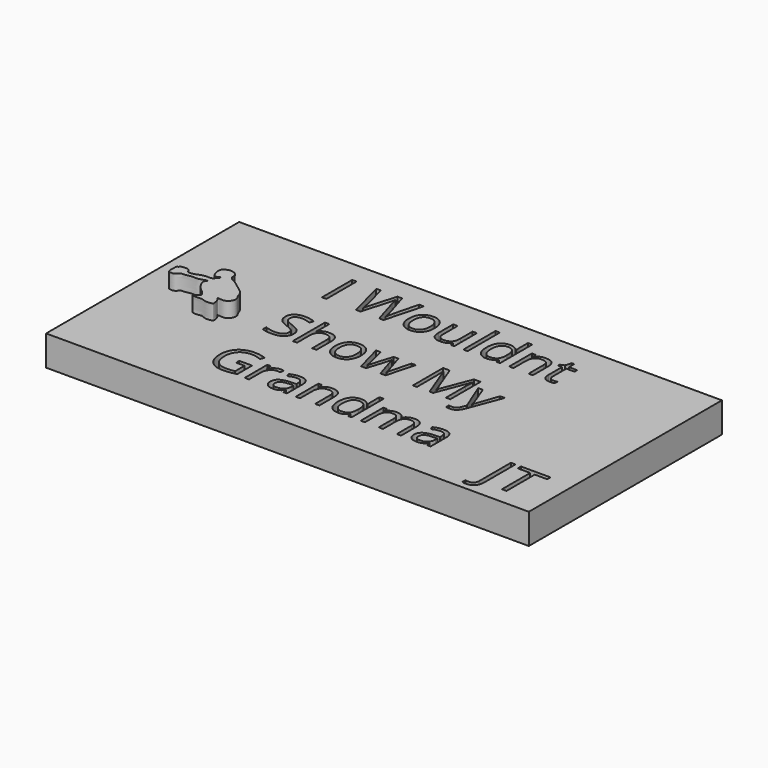
from build123d import *

# Parameters (mm, degrees)
F0_W         = 101.6
F0_H         = 50.8
F1_DEPTH     = 6.35
F2_TEXT_SIZE = 11.1437874893
F3_DEPTH     = 3.175
F4_TEXT_SIZE = 11.5956541979
F5_DEPTH     = 3.175
F7_DEPTH     = 3.175


# Not quite as in the source:
# - Text() gives the source's letters only with a copy of the font that has no kerning and outlines rounded to 1/6400 em; it was checked with that copy


with BuildPart() as f1:
    # F0 (on Top) → F1 (new body)
    with BuildSketch(Plane.XY):
        with Locations((1.0436102748, -12.8909808933)):
            Rectangle(F0_W, F0_H)
    extrude(amount=F1_DEPTH)

    # F2 (on face) → F3 (cut)
    with BuildSketch(Plane.XY.offset(6.35)):
        with Locations((-23.4671995546, 0.0636447086)):
            Text('I Wouldnt', F2_TEXT_SIZE, font='Open Sans', text_align=(TextAlign.LEFT, TextAlign.BOTTOM))
        with Locations((-23.4671995546, -15.0919062768)):
            Text('Show My', F2_TEXT_SIZE, font='Open Sans', text_align=(TextAlign.LEFT, TextAlign.BOTTOM))
        with Locations((-23.4671995546, -30.2474572623)):
            Text('Grandma', F2_TEXT_SIZE, font='Open Sans', text_align=(TextAlign.LEFT, TextAlign.BOTTOM))
    extrude(amount=-F3_DEPTH, mode=Mode.SUBTRACT)

    # F4 (on face) → F5 (cut)
    with BuildSketch(Plane.XY.offset(6.35)):
        with Locations((37.5699140131, -34.7869619727)):
            Text('JT', F4_TEXT_SIZE, font='Open Sans', text_align=(TextAlign.LEFT, TextAlign.BOTTOM))
    extrude(amount=-F5_DEPTH, mode=Mode.SUBTRACT)

    # F6 (on face) → F7 (join)
    with BuildSketch(Plane.XY.offset(6.35)):
        with BuildLine():
            add(Edge.make_bspline(
                [(-38.1303168833, -12.1464030817), (-38.316946493, -12.2069298464), (-38.4556670309, -12.2159674061), (-39.0389928869, -12.3410064962), (-39.812706995, -12.1674415845), (-41.2114169104, -12.59194698), (-41.9601470499, -12.3988371901), (-42.437010517, -13.0739388184), (-42.9595849941, -13.3882776205), (-43.5586782025, -13.309062327), (-43.8288392387, -13.2999414746), (-44.157598544, -13.0223378307), (-44.1289442843, -12.185893612), (-44.0782311075, -11.7570404612), (-44.1280417217, -10.9490263531), (-43.6482512875, -11.0103438509), (-43.7891729349, -10.7705751866), (-43.3048060572, -10.532395362), (-42.3660225836, -10.4879313303), (-41.6172761303, -10.7627556228), (-41.5950416729, -11.4429677209), (-40.7259663742, -11.5183280611), (-39.6836808018, -11.1978367036), (-38.5995973674, -10.7038706948), (-37.441166018, -10.7839163431), (-36.6191850347, -10.6613742912), (-36.4642760538, -10.1300350814), (-36.0099054285, -9.9350600118), (-35.9311626552, -9.4954912322), (-36.4194659013, -9.5581108064), (-36.5178485085, -9.8201746473), (-36.9838709459, -9.7861143723), (-37.529851152, -9.4742462715), (-38.0772211882, -7.287036148), (-36.9690859852, -6.6857934275), (-36.8699922871, -6.9393391331), (-36.6628772435, -6.7231226915), (-36.2577533517, -6.611942127), (-35.363441984, -6.7604672827), (-34.8689422251, -7.1525957855), (-34.5218728707, -7.811481285), (-34.5922251376, -8.3930239198), (-34.4489526058, -8.4653935889), (-34.1913935466, -8.9880261637), (-33.646938159, -8.9968094589), (-31.8417004696, -10.3326879226), (-29.8957191309, -11.7575187922), (-29.7075408197, -12.9935479714), (-29.1990884298, -13.5418517242), (-29.0845405883, -14.5313547928), (-29.8372999202, -15.4906855155), (-30.7738364124, -15.7587608718), (-32.0252457812, -15.4368417914), (-31.3727296309, -16.0607277656), (-31.1763513348, -16.9005418333), (-31.0913739929, -17.5893244862), (-31.3247138836, -17.70568722), (-32.8293789588, -17.9001742379), (-33.6119408094, -17.280585993), (-34.8941372032, -17.6525424411), (-36.0029992008, -17.3134002802), (-35.2036724308, -16.936679359), (-34.2501039816, -16.5238367629), (-35.4090744679, -15.2090390729), (-36.355304901, -14.5257346975), (-37.0987938745, -13.3536780956), (-37.4704305195, -12.3492894388), (-36.5163170435, -11.5294785004), (-37.7880310347, -12.0353946782), (-38.1303168833, -12.1464030817)],
                knots=[0, 0, 0, 0, 0.0107071507, 0.0233089791, 0.0392797652, 0.0604859213, 0.0752560027, 0.0902880048, 0.1040624564, 0.1173894298, 0.1264153845, 0.1370686625, 0.1526913834, 0.1654776963, 0.1798390381, 0.1892126321, 0.1957673588, 0.2073264211, 0.2250050716, 0.2398934017, 0.2525994758, 0.2674952907, 0.2862629386, 0.3055337232, 0.3246917458, 0.339878642, 0.3520374392, 0.3642110652, 0.3736560456, 0.3840959901, 0.3928749616, 0.4037117376, 0.4174022394, 0.4426935804, 0.459293658, 0.4657208648, 0.4738943866, 0.4854441438, 0.5019852742, 0.5160027755, 0.5311902422, 0.5438712607, 0.5504259607, 0.5629093031, 0.5751135105, 0.6013968753, 0.6292021137, 0.647824756, 0.6625942055, 0.6793639751, 0.6980271292, 0.7160986, 0.732523899, 0.7449434935, 0.7624922829, 0.7762541508, 0.7841258829, 0.8051423975, 0.8226408753, 0.8431057527, 0.8584517421, 0.8719110447, 0.8876817197, 0.9083167756, 0.9284511782, 0.9490862438, 0.9669541201, 0.9803626757, 1, 1, 1, 1], degree=3))
        make_face()
    extrude(amount=F7_DEPTH)


solid = f1.part
